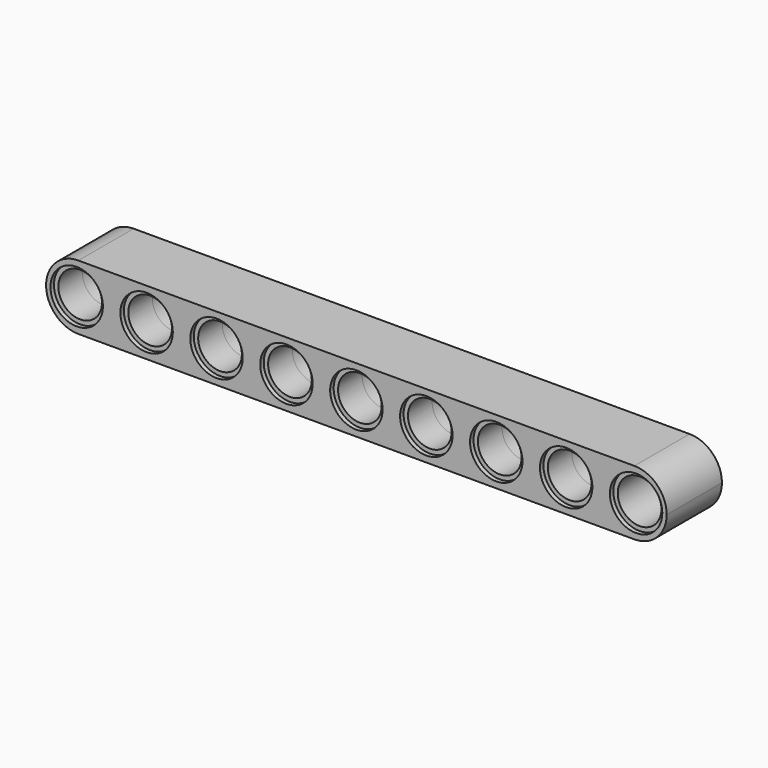
from build123d import *

# Parameters (mm, degrees)
F0_R     = 3
F1_DEPTH = 3.95
F0_R_2   = 2.499
F2_DEPTH = 3.45
F3_R     = 3.69999
F4_R     = 3.69999


# Not quite as in the source:
# - a fillet or chamfer is up to 0.001 mm smaller than in the source, because OpenCascade refuses the exact size


with BuildPart() as f1:
    # F0 (on Front) → F1 (new body, symmetric)
    with BuildSketch(Plane.XZ):
        Polygon((-35.5, 0), (0, 0), (35.5, 0), (35.5, 7.4), (-35.5, 7.4), align=None)
        with Locations((-32, 3.7)):
            Circle(F0_R, mode=Mode.SUBTRACT)
        with Locations((-24, 3.7)):
            Circle(F0_R, mode=Mode.SUBTRACT)
        with Locations((-16, 3.7)):
            Circle(F0_R, mode=Mode.SUBTRACT)
        with Locations((-8, 3.7)):
            Circle(F0_R, mode=Mode.SUBTRACT)
        with Locations((0, 3.7)):
            Circle(F0_R, mode=Mode.SUBTRACT)
        with Locations((8, 3.7)):
            Circle(F0_R, mode=Mode.SUBTRACT)
        with Locations((16, 3.7)):
            Circle(F0_R, mode=Mode.SUBTRACT)
        with Locations((24, 3.7)):
            Circle(F0_R, mode=Mode.SUBTRACT)
        with Locations((32, 3.7)):
            Circle(F0_R, mode=Mode.SUBTRACT)
    extrude(amount=F1_DEPTH, both=True)

    # F0 (on Front) → F2 (join, symmetric)
    with BuildSketch(Plane.XZ):
        with Locations((0, 3.7)):
            Circle(F0_R)
        with Locations((0, 3.7)):
            Circle(F0_R_2, mode=Mode.SUBTRACT)
        with Locations((-32, 3.7)):
            Circle(F0_R)
        with Locations((-32, 3.7)):
            Circle(F0_R_2, mode=Mode.SUBTRACT)
        with Locations((-24, 3.7)):
            Circle(F0_R)
        with Locations((-24, 3.7)):
            Circle(F0_R_2, mode=Mode.SUBTRACT)
        with Locations((-16, 3.7)):
            Circle(F0_R)
        with Locations((-16, 3.7)):
            Circle(F0_R_2, mode=Mode.SUBTRACT)
        with Locations((-8, 3.7)):
            Circle(F0_R)
        with Locations((-8, 3.7)):
            Circle(F0_R_2, mode=Mode.SUBTRACT)
        with Locations((8, 3.7)):
            Circle(F0_R)
        with Locations((8, 3.7)):
            Circle(F0_R_2, mode=Mode.SUBTRACT)
        with Locations((16, 3.7)):
            Circle(F0_R)
        with Locations((16, 3.7)):
            Circle(F0_R_2, mode=Mode.SUBTRACT)
        with Locations((24, 3.7)):
            Circle(F0_R)
        with Locations((24, 3.7)):
            Circle(F0_R_2, mode=Mode.SUBTRACT)
        with Locations((32, 3.7)):
            Circle(F0_R)
        with Locations((32, 3.7)):
            Circle(F0_R_2, mode=Mode.SUBTRACT)
    extrude(amount=F2_DEPTH, both=True)

    # F3 (radius 3.7 in the source; OpenCascade refuses exactly that, so slightly less here)
    f3_edges = [f1.edges().sort_by_distance(p)[0] for p in [
        (-35.5, 0, 7.4),
        (-35.5, 0, 0),
    ]]
    fillet(f3_edges, radius=F3_R)

    # F4 (radius 3.7 in the source; OpenCascade refuses exactly that, so slightly less here)
    f4_edges = [f1.edges().sort_by_distance(p)[0] for p in [
        (35.5, 0, 7.4),
        (35.5, 0, 0),
    ]]
    fillet(f4_edges, radius=F4_R)


solid = f1.part
